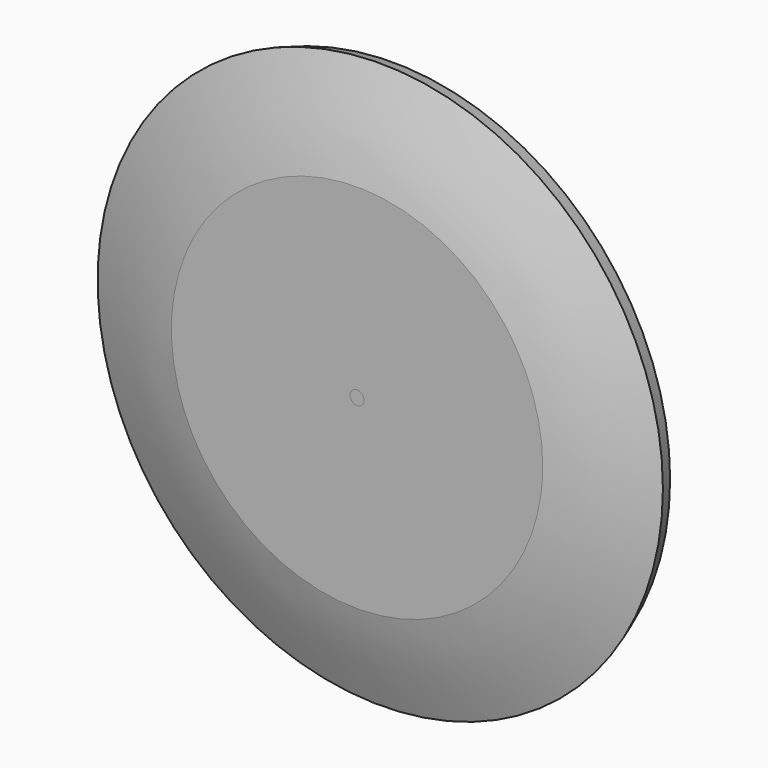
from build123d import *

# Parameters (mm, degrees)
F2_R     = 80.6344691004
F3_DEPTH = 25.4


# Not quite as in the source:
# - the dataset's text gives a spline's control points without its knots; the knots are read off the source's solid


with BuildPart() as f1:
    # F0 (on Top) → F1 (revolve)
    with BuildSketch(Plane.XY):
        with BuildLine():
            Line((-26.850635668, 3.175), (-26.850635668, 0))
            add(Edge.make_bspline(
                [(25.5485544403, 5.3778804894), (23.1985597561, 4.5465525815), (19.6566079234, 3.2860761015), (14.8833198328, 1.7743916786), (11.2721598751, 0.7764677547), (8.2307124845, 0.1023205135), (5.7773253577, -0.3142432691), (3.9218388528, -0.5583467592), (2.0706201525, -0.7249494119), (-0.3645168419, -0.8558158175), (-3.3417463146, -0.8742114936), (-6.7613578997, -0.741208201), (-9.9810989679, -0.5277370357), (-12.4586816734, -0.3421454186), (-14.2783279737, -0.2249204361), (-16.0207399212, -0.1329638728), (-18.1217352075, -0.0571073816), (-20.7029775252, -0.0128522745), (-23.5242370522, 0.000700008), (-25.6779890698, 0), (-26.850635668, 0)],
                knots=[0, 0, 0, 0, 0.125, 0.1875, 0.25, 0.3125, 0.34375, 0.375, 0.40625, 0.4375, 0.5, 0.5625, 0.625, 0.6875, 0.71875, 0.75, 0.8125, 0.875, 0.9375, 1, 1, 1, 1], degree=3))
            Line((25.5485544403, 5.3778804894), (24.4896784425, 8.3711072803))
            add(Edge.make_bspline(
                [(24.4896784425, 8.3711072803), (17.4545197529, 5.8823681377), (4.3595654098, 1.1725124121), (-13.9965163599, 3.1915448875), (-21.3583604395, 3.175), (-26.850635668, 3.175)],
                knots=[0, 0, 0, 0, 0.3736628225, 0.7071124792, 1, 1, 1, 1], degree=3))
        make_face()
    revolve(axis=Axis((-26.850635668, 1.5875, 0), (0, 1, 0)))

    # F2 (on Front) → F3 (cut)
    with BuildSketch(Plane.XZ):
        with Locations((-26.850635668, 0)):
            Circle(F2_R)
    extrude(amount=F3_DEPTH, mode=Mode.SUBTRACT)


solid = f1.part
